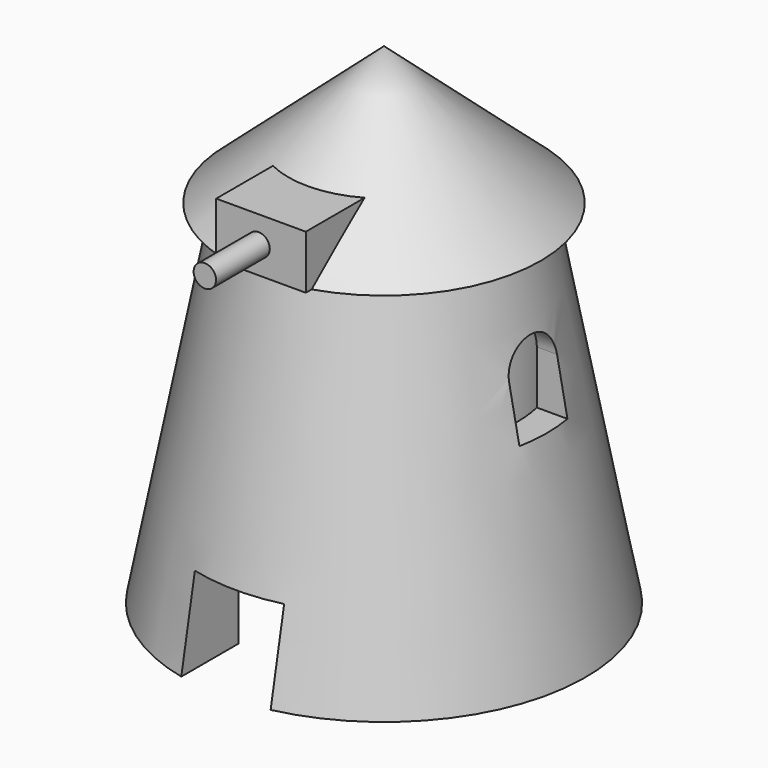
from build123d import *

# Parameters (mm, degrees)
F3_DEPTH       = 87.884
F4_R           = 37.6973348858
F5_DEPTH       = 98.044
F7_DEPTH       = 44.45
F8_R           = 3.175
F9_DEPTH       = 19.05
F11_DEPTH      = 67.564
F11_DEPTH_BACK = 62.992


with BuildPart() as f1:
    # F0 (on Front) → F1 (revolve)
    with BuildSketch(Plane.XZ):
        Polygon((0, 38.7462731748), (-38.1, 38.7462731748), (-57.15, -61.0518104742), (0, -61.0518104742), align=None)
        Polygon((-44.45, 38.7462731748), (-38.1, 38.7462731748), (0, 38.7462731748), (0, 77.8838843107), align=None)
    revolve(axis=Axis((0, 0, -11.1527686497), (0, 0, 1)))

    # F2 (on Front) → F3 (cut)
    with BuildSketch(Plane.XZ):
        Polygon((12.4711716, -36.5671299331), (0, -36.5671299331), (-12.9288284, -36.5671299331), (-12.9288284, -61.0518104742), (0, -61.0518104742), (12.4711716, -61.0518104742), align=None)
    extrude(amount=F3_DEPTH, mode=Mode.SUBTRACT)

    # F4 (on face) → F5 (cut)
    with BuildSketch(Plane(origin=(0, 0, -61.0518104742), x_dir=(1, 0, 0), z_dir=(0, 0, -1))):
        Circle(F4_R)
    extrude(amount=-F5_DEPTH, mode=Mode.SUBTRACT)

    # F6 (on Front) → F7 (join)
    with BuildSketch(Plane.XZ):
        Polygon((-12.0120554089, 38.7462731748), (0, 38.7462731748), (13.3879445911, 38.7462731748), (13.3879445911, 53.9862731748), (0, 53.9862731748), (-12.0120554089, 53.9862731748), align=None)
    extrude(amount=F7_DEPTH)

    # F8 (on face) → F9 (join)
    with BuildSketch(Plane.XZ.offset(44.45)):
        with Locations((0, 46.3662731748)):
            Circle(F8_R)
    extrude(amount=F9_DEPTH)

    # F10 (on Right) → F11 (cut, two sides)
    with BuildSketch(Plane.YZ) as f11_sk:
        with BuildLine():
            ThreePointArc((8.1476010382, 11.462922208), (-0.4339928104, 19.6117778709), (-8.7295742705, 11.1719360575))
            Line((-8.7295742705, 11.1719360575), (-8.7295742705, -3.6683375947))
            Line((-8.7295742705, -3.6683375947), (8.1476010382, -3.6683375947))
            Line((8.1476010382, -3.6683375947), (8.1476010382, 11.462922208))
        make_face()
    extrude(amount=-F11_DEPTH, mode=Mode.SUBTRACT)
    extrude(f11_sk.sketch, amount=F11_DEPTH_BACK, mode=Mode.SUBTRACT)


solid = f1.part
